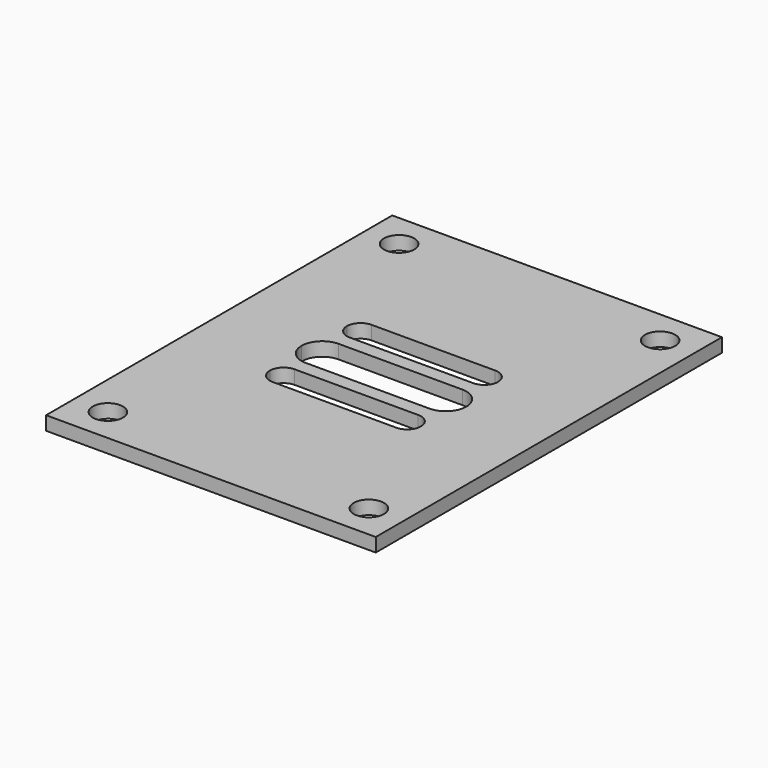
from build123d import *

# Parameters (mm, degrees)
F1_DEPTH = 2
F2_D     = 4.4
F2_DEPTH = 5
F2_TIP   = 1.3218933619


# Not quite as in the source:
# - ends of sketch curves that miss each other by under 0.0002 mm in the source are joined


with BuildPart() as f1:
    # F0 (on Top) → F1 (new body)
    with BuildSketch(Plane.XY):
        with BuildLine():
            Line((24, 0), (0, 0))
            Line((0, 0), (0, -31.5))
            Line((0, -31.5), (12, -31.5))
            ThreePointArc((12, -31.5), (12.8786796564, -29.3786796564), (15, -28.5))
            Line((15, -28.5), (24, -28.5))
            Line((24, -28.5), (24, -26.4939))
            Line((24, -26.4939), (15.0018, -26.4939))
            ThreePointArc((15.0018, -26.4939), (13.5919063065, -25.9124202759), (13.001837209, -24.506099773))
            Line((13.001837209, -24.506099773), (13.0018, -24.4939))
            ThreePointArc((13.0018, -24.4939), (13.5919063065, -23.0875797241), (15.0018, -22.5061))
            Line((15.0018, -22.5061), (24, -22.5061))
            Line((24, -22.5061), (24, 0))
        make_face()
        with BuildLine():
            Line((48, 0), (24, 0))
            Line((24, 0), (24, -22.5061))
            Line((24, -22.5061), (32.9982, -22.5061))
            ThreePointArc((32.9982, -22.5061), (34.4080936935, -23.0875797241), (34.998162791, -24.493900227))
            Line((34.998162791, -24.493900227), (34.9982, -24.5061))
            ThreePointArc((34.9982, -24.5061), (34.4080936935, -25.9124202759), (32.9982, -26.4939))
            Line((32.9982, -26.4939), (24, -26.4939))
            Line((24, -26.4939), (24, -28.5))
            Line((24, -28.5), (33, -28.5))
            ThreePointArc((33, -28.5), (35.1213203436, -29.3786796564), (36, -31.5))
            Line((36, -31.5), (48, -31.5))
            Line((48, -31.5), (48, 0))
        make_face()
        with BuildLine():
            Line((12, -31.5), (0, -31.5))
            Line((0, -31.5), (0, -63))
            Line((0, -63), (24, -63))
            Line((24, -63), (24, -40.5224670172))
            Line((24, -40.5224670172), (15, -40.5224670172))
            ThreePointArc((15, -40.5224670172), (13.5857864376, -39.9366805795), (13, -38.5224670172))
            ThreePointArc((13, -38.5224670172), (13.5857864376, -37.1082534548), (15, -36.5224670172))
            Line((15, -36.5224670172), (24, -36.5224670172))
            Line((24, -36.5224670172), (24, -34.5))
            Line((24, -34.5), (15, -34.5))
            ThreePointArc((15, -34.5), (12.8786796564, -33.6213203436), (12, -31.5))
        make_face()
        with BuildLine():
            Line((48, -63), (48, -31.5))
            Line((48, -31.5), (36, -31.5))
            ThreePointArc((36, -31.5), (35.1213203436, -33.6213203436), (33, -34.5))
            Line((33, -34.5), (24, -34.5))
            Line((24, -34.5), (24, -36.5224670172))
            Line((24, -36.5224670172), (33, -36.5224670172))
            ThreePointArc((33, -36.5224670172), (34.4142135624, -37.1082534548), (35, -38.5224670172))
            ThreePointArc((35, -38.5224670172), (34.4142135624, -39.9366805795), (33, -40.5224670172))
            Line((33, -40.5224670172), (24, -40.5224670172))
            Line((24, -40.5224670172), (24, -63))
            Line((24, -63), (48, -63))
        make_face()
    extrude(amount=F1_DEPTH)

    # F2
    with Locations(Plane(origin=(0, 0, 0), x_dir=(1, 0, 0), z_dir=(0, 0, -1))):
        with Locations((5, 5), (43, 5), (43, 58), (5, 58)):
            Hole(F2_D / 2, depth=F2_DEPTH)
            with Locations((0, 0, -(F2_DEPTH + F2_TIP / 2))):  # 118° drill point
                Cone(0, F2_D / 2, F2_TIP, mode=Mode.SUBTRACT)


solid = f1.part
